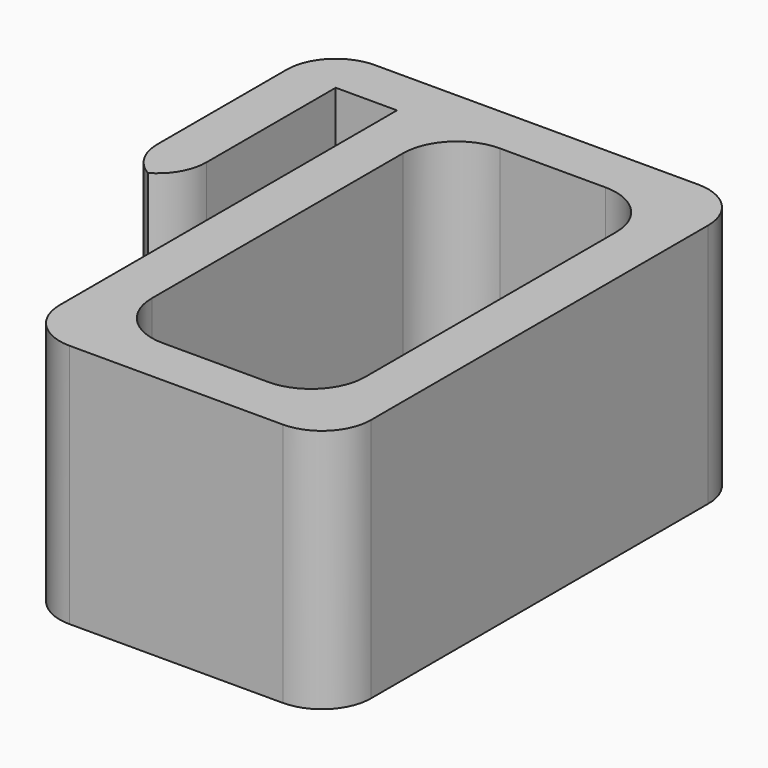
from build123d import *

# Parameters (mm, degrees)
F0_W        = 22.098
F0_H        = 43.688
F1_DEPTH    = 25.4
F2_T1_DEPTH = 50.8
F3_R        = 5.588


# Not quite as in the source:
# - a fillet or chamfer that OpenCascade refuses, or shapes differently, is made with other operations: its cross-section is extruded or revolved along the edge and cut away or added


with BuildPart() as f1:
    # F0 (on Top) → F1 (new body)
    with BuildSketch(Plane.XY):
        Polygon((21.844, -26.924), (21.844, 26.924), (-21.844, 26.924), (-21.844, 0), (-16.764, 0), (-16.764, 21.844), (-10.414, 21.844), (-10.414, -26.924), align=None)
        with Locations((5.715, 0)):
            Rectangle(F0_W, F0_H, mode=Mode.SUBTRACT)
    extrude(amount=F1_DEPTH)

    # F2: fillet of radius 5.08 on 6 edges, made by hand

    # F2_s2 → F2_t1 (cut)
    with BuildSketch(Plane.XY.offset(-12.7)):
        with BuildLine():
            ThreePointArc((-16.764, 26.924), (-20.3561024484, 25.4361024484), (-21.844, 21.844))
            Line((-21.844, 21.844), (-21.844, 26.924))
            Line((-21.844, 26.924), (-16.764, 26.924))
        make_face()
        with BuildLine():
            ThreePointArc((21.844, 21.844), (20.3561024484, 25.4361024484), (16.764, 26.924))
            Line((16.764, 26.924), (21.844, 26.924))
            Line((21.844, 26.924), (21.844, 21.844))
        make_face()
        with BuildLine():
            ThreePointArc((-5.334, -26.924), (-8.9261024484, -25.4361024484), (-10.414, -21.844))
            Line((-10.414, -21.844), (-10.414, -26.924))
            Line((-10.414, -26.924), (-5.334, -26.924))
        make_face()
        with BuildLine():
            ThreePointArc((16.764, -26.924), (20.3561024484, -25.4361024484), (21.844, -21.844))
            Line((21.844, -21.844), (21.844, -26.924))
            Line((21.844, -26.924), (16.764, -26.924))
        make_face()
        with BuildLine():
            ThreePointArc((-21.844, 0), (-18.2518975516, 1.4878975516), (-16.764, 5.08))
            Line((-16.764, 5.08), (-16.764, 0))
            Line((-16.764, 0), (-21.844, 0))
        make_face()
        with BuildLine():
            ThreePointArc((-21.844, 5.08), (-20.3561024484, 1.4878975516), (-16.764, 0))
            Line((-16.764, 0), (-21.844, 0))
            Line((-21.844, 0), (-21.844, 5.08))
        make_face()
    extrude(amount=F2_T1_DEPTH, mode=Mode.SUBTRACT)

    # F3
    f3_edges = [f1.edges().sort_by_distance(p)[0] for p in [
        (-5.334, -21.844, 12.7),
        (16.764, -21.844, 12.7),
        (16.764, 21.844, 12.7),
        (-5.334, 21.844, 12.7),
    ]]
    fillet(f3_edges, radius=F3_R)


solid = f1.part
